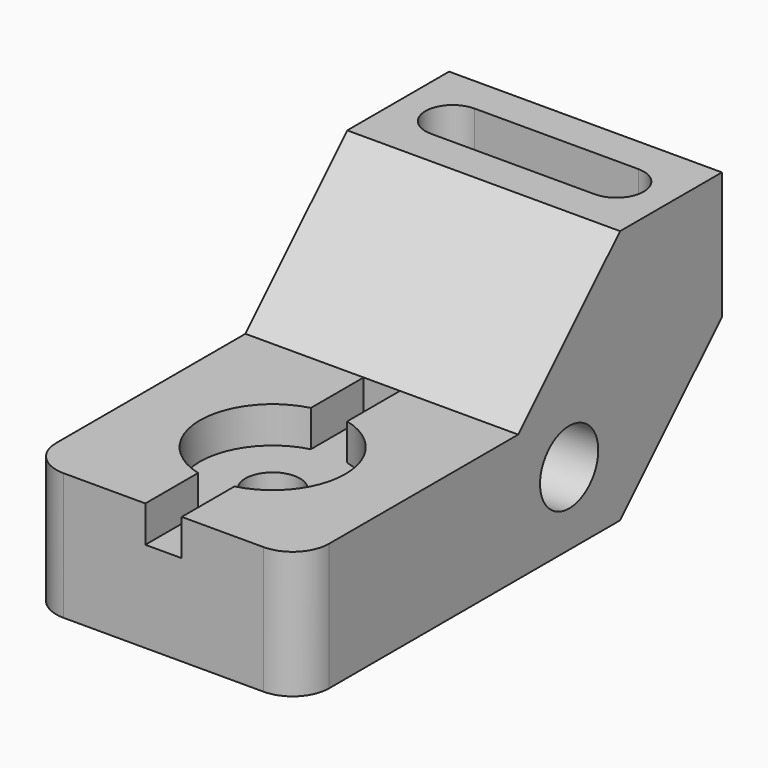
from build123d import *

# Parameters (mm, degrees)
F0_W           = 147.32
F0_H           = 71.12
F1_DEPTH       = 76.2
F3_DEPTH       = 76.201
F5_DEPTH       = 27.94
F7_D           = 15.24
F7_CBORE_D     = 40.64
F7_CBORE_DEPTH = 10.16
F9_DEPTH       = 10.16
F11_D          = 20.32
F12_R          = 10.16


with BuildPart() as f1:
    # F0 (on Right) → F1 (new body)
    with BuildSketch(Plane.YZ):
        with Locations((73.66, 35.56)):
            Rectangle(F0_W, F0_H)
    extrude(amount=F1_DEPTH)

    # F2 (on face) → F3 (cut, through all)
    with BuildSketch(Plane.YZ.offset(76.2)):
        Polygon((0, 71.12), (0, 35.56), (76.2, 35.56), (111.76, 71.12), align=None)
        Polygon((147.32, 35.56), (111.76, 0), (147.32, 0), align=None)
    extrude(amount=-F3_DEPTH, mode=Mode.SUBTRACT)

    # F4 (on face) → F5 (cut)
    with BuildSketch(Plane.XY.offset(71.12)):
        with BuildLine():
            ThreePointArc((15.24, 137.16), (7.62, 129.54), (15.24, 121.92))
            Line((15.24, 121.92), (60.96, 121.92))
            ThreePointArc((60.96, 121.92), (68.58, 129.54), (60.96, 137.16))
            Line((60.96, 137.16), (15.24, 137.16))
        make_face()
    extrude(amount=-F5_DEPTH, mode=Mode.SUBTRACT)

    # F7 (through all)
    with Locations(Plane.XY.offset(35.56)):
        with Locations((38.1, 38.1)):
            CounterBoreHole(F7_D / 2, F7_CBORE_D / 2, F7_CBORE_DEPTH)

    # F8 (on face) → F9 (cut)
    with BuildSketch(Plane.XY.offset(35.56)):
        with BuildLine():
            Line((43.18, 76.2), (33.02, 76.2))
            Line((33.02, 76.2), (33.02, 57.7747553987))
            ThreePointArc((33.02, 57.7747553987), (38.1, 58.42), (43.18, 57.7747553987))
            Line((43.18, 57.7747553987), (43.18, 76.2))
        make_face()
        with BuildLine():
            ThreePointArc((43.18, 18.4252446013), (38.1, 17.78), (33.02, 18.4252446013))
            Line((33.02, 18.4252446013), (33.02, 0))
            Line((33.02, 0), (43.18, 0))
            Line((43.18, 0), (43.18, 18.4252446013))
        make_face()
    extrude(amount=-F9_DEPTH, mode=Mode.SUBTRACT)

    # F11 (through all)
    with Locations(Plane.YZ.offset(76.2)):
        with Locations((93.98, 20.32)):
            Hole(F11_D / 2)

    # F12
    f12_edges = [f1.edges().sort_by_distance(p)[0] for p in [
        (0, 0, 17.78),
        (76.2, 0, 17.78),
    ]]
    fillet(f12_edges, radius=F12_R)


solid = f1.part
